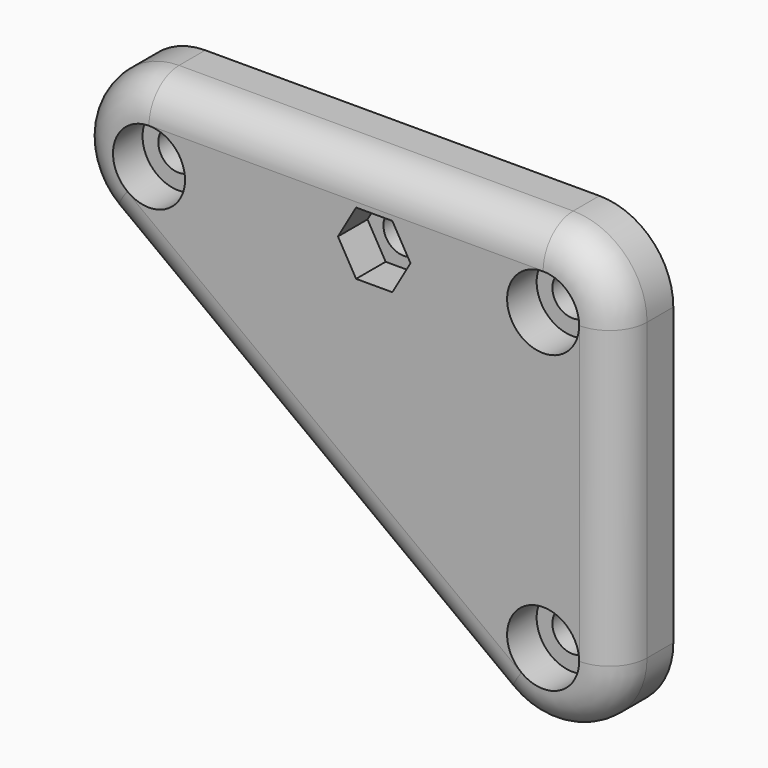
from build123d import *

# Parameters (mm, degrees)
F1_DEPTH       = 9.525
F2_D           = 5.5
F2_CBORE_D     = 9.75
F2_CBORE_DEPTH = 5
F3_R           = 5.08
F4_DEPTH       = 5
F5_D           = 5.5


# Not quite as in the source:
# - a feature names something its author has since deleted; it is built from what else it names


with BuildPart() as f1:
    # F0 (on Front) → F1 (new body)
    with BuildSketch(Plane.XZ):
        with BuildLine():
            Line((10, -40), (10, 0))
            ThreePointArc((10, 0), (7.0710678119, 7.0710678119), (0, 10))
            Line((0, 10), (-53.34, 10))
            ThreePointArc((-53.34, 10), (-62.826927837, 3.1619930765), (-59.3395200276, -8.0003599568))
            Line((-59.3395200276, -8.0003599568), (-5.9995200276, -48.0003599568))
            ThreePointArc((-5.9995200276, -48.0003599568), (4.4724042597, -48.9441377526), (10, -40))
        make_face()
        Polygon((-17.9525227119, 0), (-20.4062613559, -4.25), (-25.3137386441, -4.25), (-27.7674772881, 0), (-25.3137386441, 4.25), (-20.4062613559, 4.25), align=None, mode=Mode.SUBTRACT)
        Polygon((-25.3137386441, -4.25), (-20.4062613559, -4.25), (-17.9525227119, 0), (-20.4062613559, 4.25), (-25.3137386441, 4.25), (-27.7674772881, 0), align=None)
    extrude(amount=-F1_DEPTH)

    # F2 (through all)
    with Locations(Plane.XZ):
        with Locations((0, 0), (0, -40), (-53.34, 0)):
            CounterBoreHole(F2_D / 2, F2_CBORE_D / 2, F2_CBORE_DEPTH)

    # F3
    f3_edges = [f1.edges().sort_by_distance(p)[0] for p in [
        (-26.67, 0, 10),
    ]]
    fillet(f3_edges, radius=F3_R)

    # F0 (on Front) → F4 (cut)
    with BuildSketch(Plane.XZ):
        Polygon((-25.3137386441, -4.25), (-20.4062613559, -4.25), (-17.9525227119, 0), (-20.4062613559, 4.25), (-25.3137386441, 4.25), (-27.7674772881, 0), align=None)
    extrude(amount=-F4_DEPTH, mode=Mode.SUBTRACT)

    # F5 (through all)
    with Locations(Plane.XZ):
        with Locations((-22.86, 0)):
            Hole(F5_D / 2)


solid = f1.part
